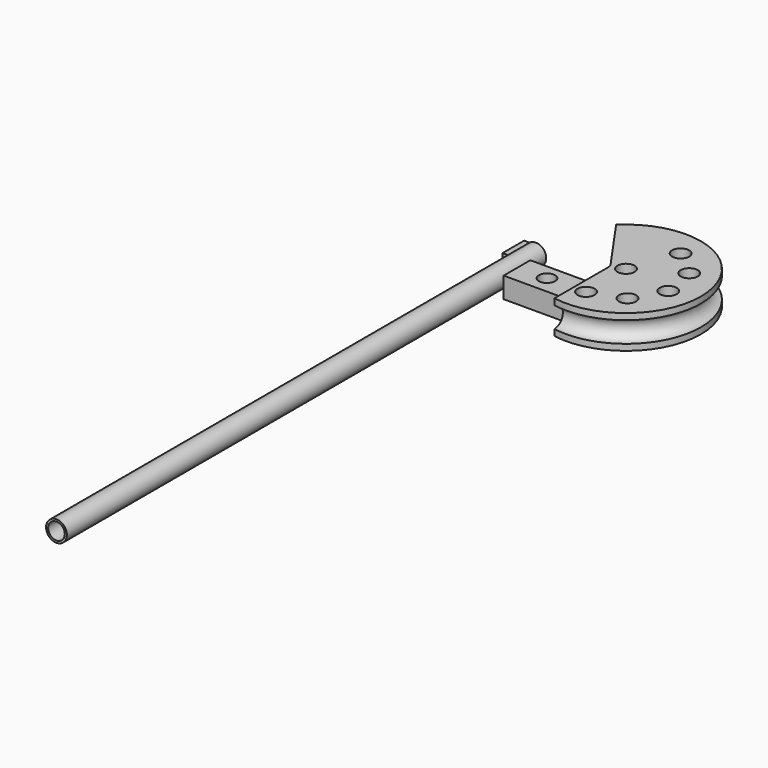
from build123d import *

# Parameters (mm, degrees)
F0_R            = 13.0937
F1_DEPTH        = 25.4
F3_R            = 13.0937
F4_DEPTH        = 63.5
F4_COPIES_COUNT = 5
F4_COPIES_ANGLE = 160
F5_R            = 15.875
F7_W            = 95.25
F7_H            = 50.8
F7_R            = 12.3737085095
F8_DEPTH        = 15.875
F9_R            = 12.7
F10_R           = 15.875
F10_R_2         = 12.7
F11_DEPTH       = 914.4
F12_W           = 10.9309703112
F12_H           = 41.1224626005
F13_DEPTH       = 12.7


# Not quite as in the source:
# - a pattern or mirror of a feature is missing from the dataset's text; its kind, count and spacing are read off the source's solid


with BuildPart() as f1:
    # F0 (on Top) → F1 (new body, symmetric)
    with BuildSketch(Plane.XY):
        with BuildLine():
            Line((-19.05, -6.0064419281), (-19.05, -112.701319868))
            ThreePointArc((-19.05, -112.701319868), (109.0098474705, 34.3706728833), (-80.2476678657, 81.3928854515))
            Line((-80.2476678657, 81.3928854515), (-19.05, -6.0064419281))
        make_face()
        Circle(F0_R, mode=Mode.SUBTRACT)
    extrude(amount=F1_DEPTH, both=True)

    # F3 (on Top) → F4 (cut, symmetric)
    with BuildSketch(Plane.XY):
        with Locations((0, -76.2)):
            Circle(F3_R)
    f4 = extrude(amount=F4_DEPTH, both=True, mode=Mode.SUBTRACT)

    # F4_copies: F4 ×5 about axis
    f4_copies_axis = Axis((0, 0, 0), (0, 0, 1))
    for i in range(1, F4_COPIES_COUNT):
        add(f4.rotate(f4_copies_axis, i * F4_COPIES_ANGLE / (F4_COPIES_COUNT - 1)), mode=Mode.SUBTRACT)

    # F5 (on Front) → F6 (revolve, cut)
    with BuildSketch(Plane.XZ):
        with Locations((114.3, 0)):
            Circle(F5_R)
    revolve(axis=Axis((0, 0, 0), (0, 0, -1)), mode=Mode.SUBTRACT)

    # F7 (on Top) → F8 (join, symmetric)
    with BuildSketch(Plane.XY):
        with Locations((-66.675, -65.076319868)):
            Rectangle(F7_W, F7_H)
        with Locations((-69.85, -63.5)):
            Circle(F7_R, mode=Mode.SUBTRACT)
    extrude(amount=F8_DEPTH, both=True)

    # F9
    f9_edges = [f1.edges().sort_by_distance(p)[0] for p in [
        (-19.05, -6.006442, 0),
    ]]
    fillet(f9_edges, radius=F9_R)


with BuildPart() as f11:
    # F10 (on Front) → F11 (new body)
    with BuildSketch(Plane.XZ):
        with Locations((-137.6804935392, 0)):
            Circle(F10_R)
        with Locations((-137.6804935392, 0)):
            Circle(F10_R_2, mode=Mode.SUBTRACT)
    extrude(amount=F11_DEPTH)

    # F12 (on Top) → F13 (join, symmetric)
    with BuildSketch(Plane.XY):
        with Locations((-150.0622108579, -20.5612313002)):
            Rectangle(F12_W, F12_H)
    extrude(amount=F13_DEPTH, both=True)


solid = Compound([f1.part, f11.part])
